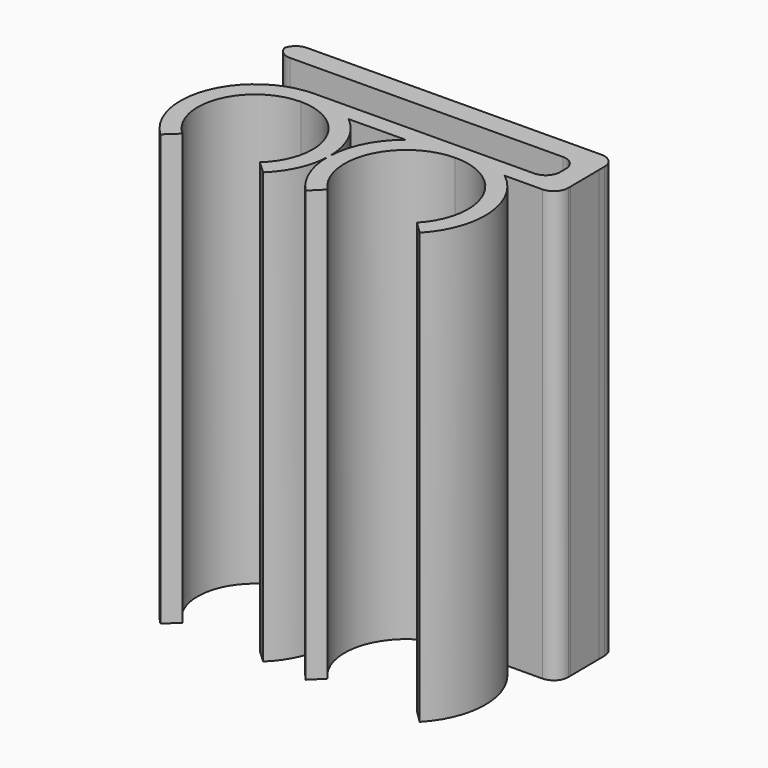
from build123d import *

# Parameters (mm, degrees)
F1_DEPTH    = 30
F2_T1_DEPTH = 30
F2_T3_DEPTH = 35


# Not quite as in the source:
# - a fillet or chamfer that OpenCascade refuses, or shapes differently, is made with other operations: its cross-section is extruded or revolved along the edge and cut away or added
# - ends of sketch curves that miss each other by under 0.0002 mm in the source are joined


with BuildPart() as f1:
    # F0 (on Top) → F1 (new body)
    with BuildSketch(Plane.XY):
        with BuildLine():
            ThreePointArc((0.0108101467, 3.9999853926), (3.7311619501, 1.441676282), (2.6975556514, -2.9535052916))
            Line((2.6975556514, -2.9535052916), (3.5790398152, -3.7723300494))
            ThreePointArc((3.5790398152, -3.7723300494), (4.7376169007, -2.1435918693), (5.1962235425, -0.1981436252))
            ThreePointArc((5.1962235425, -0.1981436252), (5.1972192437, -0.0990548017), (5.2, 0))
            ThreePointArc((5.2, 0), (4.6973944029, 2.2303555374), (3.2867362218, 4.0295613915))
            Line((3.2867362218, 4.0295613915), (0.0108101467, 3.9999853926))
        make_face()
        with BuildLine():
            ThreePointArc((-2.6975556514, -2.9535052916), (-3.7272521414, 1.4517546193), (0.0108101467, 3.9999853926))
            Line((0.0108101467, 3.9999853926), (3.2867362218, 4.0295613915))
            ThreePointArc((3.2867362218, 4.0295613915), (1.7444599113, 4.8986589612), (0, 5.2))
            ThreePointArc((0, 5.2), (-4.8299128489, 1.9266400472), (-3.5790398152, -3.7723300494))
            Line((-3.5790398152, -3.7723300494), (-2.6975556514, -2.9535052916))
        make_face()
        with BuildLine():
            ThreePointArc((0, 5.2), (1.7444599113, 4.8986589612), (3.2867362218, 4.0295613915))
            Line((3.2867362218, 4.0295613915), (7.2283371129, 4.065071131))
            ThreePointArc((7.2283371129, 4.065071131), (8.8329374117, 4.9709020374), (10.646673336, 5.2959154939))
            Line((10.646673336, 5.2959154939), (0, 5.2))
        make_face()
        with BuildLine():
            ThreePointArc((5.2, 0), (5.1972192437, -0.0990548017), (5.1962235425, -0.1981436252))
            ThreePointArc((5.1962235425, -0.1981436252), (5.1990557999, -0.099089805), (5.2, 0))
        make_face()
        with BuildLine():
            ThreePointArc((5.2, 0), (5.1990557999, -0.099089805), (5.1962235425, -0.1981436252))
            ThreePointArc((5.1962235425, -0.1981436252), (5.5915030666, -2.2512643656), (6.7244861035, -4.0085065559))
            Line((6.7244861035, -4.0085065559), (7.5779271506, -3.1646460444))
            ThreePointArc((7.5779271506, -3.1646460444), (6.7375812297, 1.4751784497), (10.6574836162, 4.0959641875))
            Line((10.6574836162, 4.0959641875), (7.2283371129, 4.065071131))
            ThreePointArc((7.2283371129, 4.065071131), (5.7748395568, 2.2517463212), (5.2, 0))
        make_face()
        with BuildLine():
            ThreePointArc((10.646673336, 5.2959154939), (8.8329374117, 4.9709020374), (7.2283371129, 4.065071131))
            Line((7.2283371129, 4.065071131), (10.6574836162, 4.0959641875))
            Line((10.6574836162, 4.0959641875), (14.0866300839, 4.1268572436))
            ThreePointArc((14.0866300839, 4.1268572436), (12.4659704087, 5.0036318817), (10.646673336, 5.2959154939))
        make_face()
        with BuildLine():
            Line((16.1859897918, 5.345818995), (10.646673336, 5.2959154939))
            ThreePointArc((10.646673336, 5.2959154939), (12.4659704087, 5.0036318817), (14.0866300839, 4.1268572436))
            Line((14.0866300839, 4.1268572436), (17.6967392423, 4.1593805861))
            Line((17.6967392423, 4.1593805861), (17.6859289245, 5.3593318922))
            Line((17.6859289245, 5.3593318922), (16.1859897918, 5.345818995))
        make_face()
        with BuildLine():
            Line((14.0866300839, 4.1268572436), (10.6574836162, 4.0959641875))
            ThreePointArc((10.6574836162, 4.0959641875), (14.6395734892, 1.510772092), (13.8145139904, -3.1646460444))
            Line((13.8145139904, -3.1646460444), (14.6679550375, -4.0085065559))
            ThreePointArc((14.6679550375, -4.0085065559), (16.1822325131, 0.1881501089), (14.0866300839, 4.1268572436))
        make_face()
        Polygon((16.1634682964, 7.8457175493), (16.1859897918, 5.345818995), (17.6859289245, 5.3593318922), (17.6634074291, 7.8592304466), align=None)
        Polygon((-0.0225214954, 7.6998985544), (16.1634682964, 7.8457175493), (17.6634074291, 7.8592304466), (17.6498945318, 9.3591695792), (-0.0360343926, 9.199837687), (-4.7136558579, 9.1576971649), (-4.7001429606, 7.6577580323), align=None)
    extrude(amount=F1_DEPTH)

    # F2: fillet of radius 1 on 6 edges, made by hand

    # F2_s2 → F2_t1 (join)
    with BuildSketch(Plane.XY):
        with BuildLine():
            ThreePointArc((15.1635088747, 7.8367089512), (15.87322552, 7.5501976583), (16.1724768946, 6.8457581276))
            Line((16.1724768946, 6.8457581276), (16.1634682964, 7.8457175493))
            Line((16.1634682964, 7.8457175493), (15.1635088747, 7.8367089512))
        make_face()
        with BuildLine():
            ThreePointArc((16.1769811937, 6.3457784167), (15.8904699008, 5.6360617714), (15.1860303701, 5.3368103968))
            Line((15.1860303701, 5.3368103968), (16.1859897918, 5.345818995))
            Line((16.1859897918, 5.345818995), (16.1769811937, 6.3457784167))
        make_face()
    extrude(amount=F2_T1_DEPTH)

    # F2_s4 → F2_t3 (cut)
    with BuildSketch(Plane.XY.offset(-2.5)):
        with BuildLine():
            ThreePointArc((16.6967798205, 4.1503719879), (17.4012193512, 4.4496233625), (17.6877306441, 5.1593400078))
            Line((17.6877306441, 5.1593400078), (17.6967392423, 4.1593805861))
            Line((17.6967392423, 4.1593805861), (16.6967798205, 4.1503719879))
        make_face()
        with BuildLine():
            ThreePointArc((17.65890313, 8.3592101575), (17.3596517554, 9.0636496882), (16.6499351101, 9.3501609811))
            Line((16.6499351101, 9.3501609811), (17.6498945318, 9.3591695792))
            Line((17.6498945318, 9.3591695792), (17.65890313, 8.3592101575))
        make_face()
        with BuildLine():
            ThreePointArc((-3.7136964361, 9.1667057631), (-4.4181359668, 8.8674543885), (-4.7046472597, 8.1577377432))
            Line((-4.7046472597, 8.1577377432), (-4.7136558579, 9.1576971649))
            Line((-4.7136558579, 9.1576971649), (-3.7136964361, 9.1667057631))
        make_face()
        with BuildLine():
            ThreePointArc((-4.7091515588, 8.657717454), (-4.4099001842, 7.9532779233), (-3.7001835389, 7.6667666304))
            Line((-3.7001835389, 7.6667666304), (-4.7001429606, 7.6577580323))
            Line((-4.7001429606, 7.6577580323), (-4.7091515588, 8.657717454))
        make_face()
    extrude(amount=F2_T3_DEPTH, mode=Mode.SUBTRACT)


solid = f1.part
